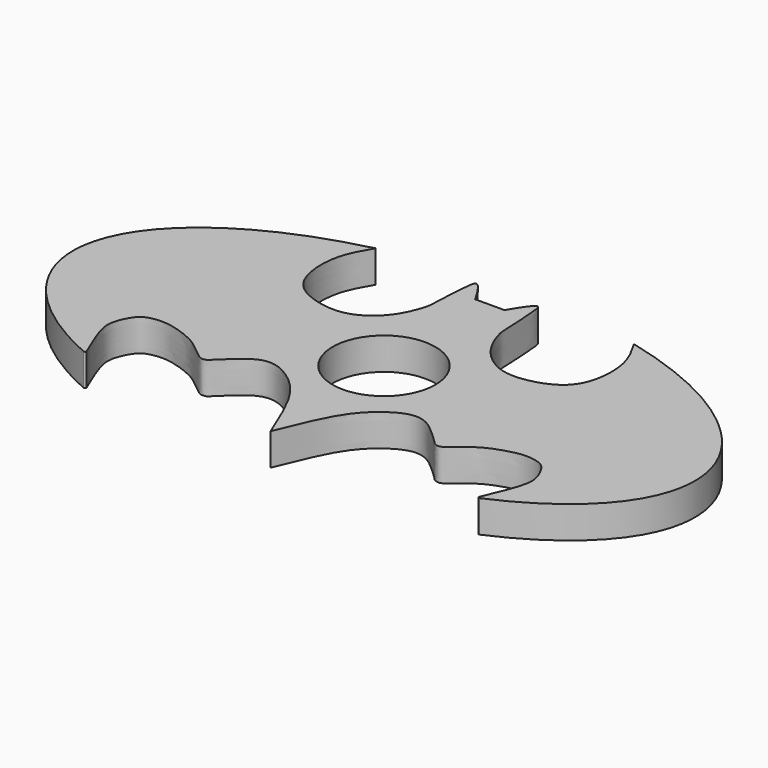
from build123d import *

# Parameters (mm, degrees)
F0_R     = 8
F1_DEPTH = 5
F3_DEPTH = 4


with BuildPart() as f1:
    # F0 (on Top) → F1 (new body)
    with BuildSketch(Plane.XY):
        with BuildLine():
            add(Edge.make_bspline(
                [(-20.1322957873, 25.53460747), (-21.0725770911, 23.9520868943), (-23.0675364795, 20.5945126588), (-22.4083503956, 12.5748714923), (-17.2545951615, 9.8940808299), (-11.7086679234, 9.3422404959), (-7.114333286, 13.0419839582), (-5.6318764107, 17.419362352), (-5.5542005863, 18.4921153575), (-5.3315524161, 24.6973197099), (-4.9661057562, 25.9294604037), (-4.5074860116, 25.9467043834), (-3.4902695158, 24.6726371533), (-2.7201798677, 23.361339468), (-2.2836024873, 22.6179417223)],
                knots=[0, 0, 0, 0, 0.1081257875, 0.2294064064, 0.3330379483, 0.4368181362, 0.544679837, 0.6371461796, 0.6891819735, 0.8016006001, 0.8496450245, 0.8727865852, 0.9278804753, 1, 1, 1, 1], degree=3))
            add(Edge.make_bspline(
                [(-20.1322957873, 25.53460747), (-90.5536915685, 8.5128706396), (-30.9104166947, -17.8634751536)],
                knots=[5.141586245, 5.141586245, 5.141586245, 7.1638946044, 7.1638946044, 7.1638946044], degree=2, weights=[1, 0.5308829712, 1]))
            ThreePointArc((-30.9104166947, -17.8634751536), (-30.6891133476, -17.8229854876), (-30.6454839702, -17.602279661))
            Line((-30.6454839702, -17.602279661), (-31.0767631014, -16.5883528518))
            add(Edge.make_bspline(
                [(0, -20.0992897153), (-1.3823299374, -16.6632151248), (-3.7259810905, -10.8375725204), (-7.5260810857, -7.3540536255), (-10.2155748152, -5.9585527548), (-12.159885229, -5.9007804143), (-13.9277435294, -6.6856686943), (-15.8876446758, -8.4566903444), (-17.2027866447, -9.625962135), (-17.6119279245, -10.2090003219), (-18.205738536, -10.3912681874), (-18.8799205861, -10.3620367326), (-20.2756503106, -9.1882203841), (-22.5170394795, -7.2842527027), (-25.5839259266, -6.1758196411), (-28.0957601751, -5.5861032814), (-30.5977671217, -5.9574582263), (-31.8337397225, -6.9177842225), (-32.9574722494, -9.2281070864), (-33.2056830629, -11.4377087655), (-31.7142961508, -15.0797440223), (-31.1854537564, -16.3327778446), (-31.0767631014, -16.5883528518)],
                knots=[0, 0, 0, 0, 0.1032899111, 0.175121375, 0.2297330056, 0.2731452478, 0.317504144, 0.3708234335, 0.4136208246, 0.4398804052, 0.4640120942, 0.4891444143, 0.531502959, 0.5878668134, 0.6462452968, 0.6987102959, 0.7485485888, 0.788300273, 0.8383671978, 0.8874172647, 0.9561263015, 0.9764684836, 0.9764684836, 0.9764684836, 0.9764684836], degree=3))
            add(Edge.make_bspline(
                [(0, -20.0992897153), (1.3823299374, -16.6632151248), (3.7259810905, -10.8375725204), (7.5260810857, -7.3540536255), (10.2155748152, -5.9585527548), (12.159885229, -5.9007804143), (13.9277435294, -6.6856686943), (15.8876446758, -8.4566903444), (17.2027866447, -9.625962135), (17.6119279245, -10.2090003219), (18.205738536, -10.3912681874), (18.8799205861, -10.3620367326), (20.2756503106, -9.1882203841), (22.5170394795, -7.2842527027), (25.5839259266, -6.1758196411), (28.0957601751, -5.5861032814), (30.5977671217, -5.9574582263), (31.8337397225, -6.9177842225), (32.9574722494, -9.2281070864), (33.2056830629, -11.4377087655), (31.7142961508, -15.0797440223), (31.1854537564, -16.3327778446), (31.0767631014, -16.5883528518)],
                knots=[0, 0, 0, 0, 0.1032899111, 0.175121375, 0.2297330056, 0.2731452478, 0.317504144, 0.3708234335, 0.4136208246, 0.4398804052, 0.4640120942, 0.4891444143, 0.531502959, 0.5878668134, 0.6462452968, 0.6987102959, 0.7485485888, 0.788300273, 0.8383671978, 0.8874172647, 0.9561263015, 0.9764684836, 0.9764684836, 0.9764684836, 0.9764684836], degree=3))
            Line((31.0767631014, -16.5883528518), (30.6113448061, -17.7075706361))
            ThreePointArc((30.6113448061, -17.7075706361), (30.6559562722, -17.9271357895), (30.8763370515, -17.9675257836))
            add(Edge.make_bspline(
                [(30.876337032, -17.9675257922), (90.5643788989, 8.2077761409), (20.1726411379, 25.4667009928)],
                knots=[2.2621161258, 2.2621161258, 2.2621161258, 4.2844215213, 4.2844215213, 4.2844215213], degree=2, weights=[1, 0.5308842271, 1]))
            add(Edge.make_bspline(
                [(20.1726411379, 25.4667009928), (21.0993637505, 23.9067183821), (23.0644753961, 20.5572715955), (22.4083503956, 12.5748714923), (17.2545951615, 9.8940808299), (11.7086679234, 9.3422404959), (7.114333286, 13.0419839582), (5.6318764107, 17.419362352), (5.5542005863, 18.4921153575), (5.3315524161, 24.6973197099), (4.9661057562, 25.9294604037), (4.5074860116, 25.9467043834), (3.4902695158, 24.6726371533), (2.7201798677, 23.361339468), (2.2836024873, 22.6179417223)],
                knots=[0.0015465389, 0.0015465389, 0.0015465389, 0.0015465389, 0.1081257875, 0.2294064064, 0.3330379483, 0.4368181362, 0.544679837, 0.6371461796, 0.6891819735, 0.8016006001, 0.8496450245, 0.8727865852, 0.9278804753, 1, 1, 1, 1], degree=3))
            Line((2.2836024873, 22.6179417223), (0, 22.6179417223))
            Line((0, 22.6179417223), (-2.2836024873, 22.6179417223))
        make_face()
        with Locations((0, 2)):
            Circle(F0_R, mode=Mode.SUBTRACT)
    extrude(amount=F1_DEPTH)

    # F2 (on face) → F3 (join)
    with BuildSketch(Plane.XY.offset(5)):
        Polygon((4.1170143522, 20.9352653474), (-3.8109705783, 21.1286321282), (-7.0981839672, 9.9134324118), (-1.6839501914, 10.880259797), (3.0535049736, 10.5902114883), (6.9208149798, 9.3333357945), (5.8573042043, 13.5873770341), align=None)
        Polygon((3.9236498997, -7.5861448422), (-3.0375095084, -7.4894623831), (-3.4242400434, -8.843020536), (0.3463879693, -15.2240833268), align=None)
    extrude(amount=-F3_DEPTH)


solid = f1.part
